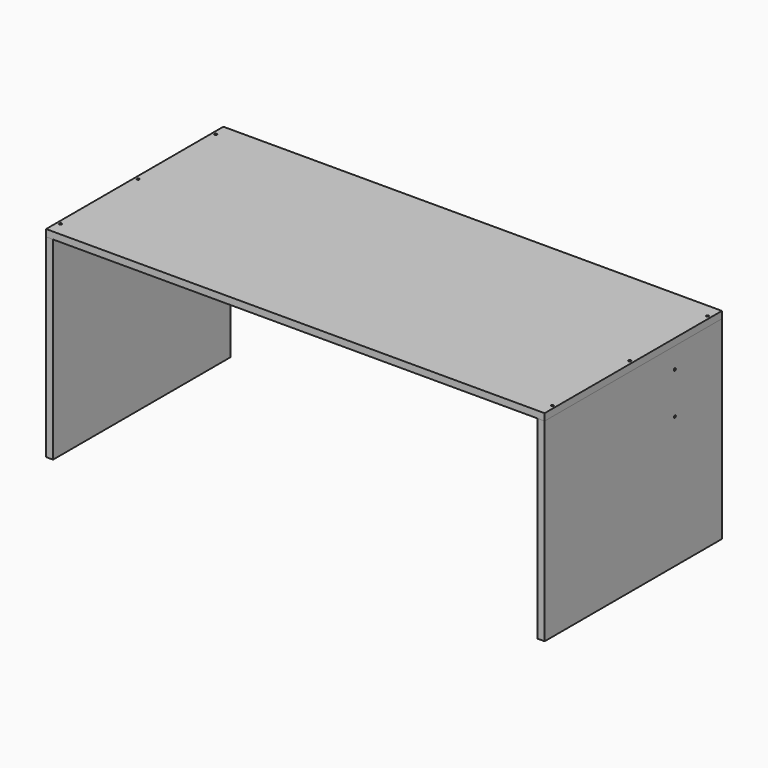
from build123d import *

# Parameters (mm, degrees)
F1_DEPTH          = 800
F0_W              = 25
F0_H              = 700
F2_DEPTH          = 800
F3_W              = 1750
F3_H              = 25
F4_DEPTH          = 300
F6_D              = 4
F6_DEPTH          = 50
F6_CSINK_D        = 8.96
F6_CSINK_ANGLE    = 90
F6_TIP            = 1.2017212381
F6_2_D            = 4
F6_2_DEPTH        = 50
F6_2_CSINK_D      = 8.96
F6_2_CSINK_ANGLE  = 90
F6_2_TIP          = 1.2017212381
F6_3_D            = 4
F6_3_DEPTH        = 50
F6_3_CSINK_D      = 8.96
F6_3_CSINK_ANGLE  = 90
F6_3_TIP          = 1.2017212381
F8_D              = 4
F8_DEPTH          = 40
F8_CSINK_D        = 8.96
F8_CSINK_ANGLE    = 90
F8_TIP            = 1.2017212381
F8_2_D            = 4
F8_2_DEPTH        = 40
F8_2_CSINK_D      = 8.96
F8_2_CSINK_ANGLE  = 90
F8_2_TIP          = 1.2017212381
F10_D             = 4
F10_DEPTH         = 40
F10_CSINK_D       = 8.96
F10_CSINK_ANGLE   = 90
F10_TIP           = 1.2017212381
F10_2_D           = 4
F10_2_DEPTH       = 40
F10_2_CSINK_D     = 8.96
F10_2_CSINK_ANGLE = 90
F10_2_TIP         = 1.2017212381
F12_D             = 3
F12_DEPTH         = 1
F12_TIP           = 0.9012909285
F12_2_D           = 3
F12_2_DEPTH       = 1
F12_2_TIP         = 0.9012909285


# Not quite as in the source:
# - a feature names something its author has since deleted; it is built from what else it names


with BuildPart() as f1:
    # F0 (on Front) → F1 (new body)
    with BuildSketch(Plane.XZ):
        Polygon((0, 25), (0, 0), (25, 0), (1775, 0), (1800, 0), (1800, 25), align=None)
    extrude(amount=-F1_DEPTH)

    # F6
    with Locations(Plane.XY.offset(25)):
        with Locations((12.5, 750), (12.5, 400), (12.5, 50), (1787.5, 750), (1787.5, 400), (1787.5, 50)):
            CounterSinkHole(F6_D / 2, F6_CSINK_D / 2, depth=F6_DEPTH, counter_sink_angle=F6_CSINK_ANGLE)
            with Locations((0, 0, -(F6_DEPTH + F6_TIP / 2))):  # 118° drill point
                Cone(0, F6_D / 2, F6_TIP, mode=Mode.SUBTRACT)


with BuildPart() as f2:
    # F0 (on Front) → F2 (new body)
    with BuildSketch(Plane.XZ):
        with Locations((12.5, -350)):
            Rectangle(F0_W, F0_H)
    extrude(amount=-F2_DEPTH)

    # F6#2
    with Locations(Plane.XY.offset(25)):
        with Locations((12.5, 750), (12.5, 400), (12.5, 50), (1787.5, 750), (1787.5, 400), (1787.5, 50)):
            CounterSinkHole(F6_2_D / 2, F6_2_CSINK_D / 2, depth=F6_2_DEPTH, counter_sink_angle=F6_2_CSINK_ANGLE)
            with Locations((0, 0, -(F6_2_DEPTH + F6_2_TIP / 2))):  # 118° drill point
                Cone(0, F6_2_D / 2, F6_2_TIP, mode=Mode.SUBTRACT)

    # F8
    with Locations(Plane(origin=(0, 0, 0), x_dir=(0, -1, 0), z_dir=(-1, 0, 0))):
        with Locations((-587.5, -75), (-587.5, -225)):
            CounterSinkHole(F8_D / 2, F8_CSINK_D / 2, depth=F8_DEPTH, counter_sink_angle=F8_CSINK_ANGLE)
            with Locations((0, 0, -(F8_DEPTH + F8_TIP / 2))):  # 118° drill point
                Cone(0, F8_D / 2, F8_TIP, mode=Mode.SUBTRACT)

    # F12
    with Locations(Plane(origin=(0, 0, -700), x_dir=(1, 0, 0), z_dir=(0, 0, -1))):
        with Locations((1787.5, -30), (1787.5, -770), (12.5, -30), (12.5, -770)):
            Hole(F12_D / 2, depth=F12_DEPTH)
            with Locations((0, 0, -(F12_DEPTH + F12_TIP / 2))):  # 118° drill point
                Cone(0, F12_D / 2, F12_TIP, mode=Mode.SUBTRACT)


with BuildPart() as f2b:
    # F0 (on Front) → F2, piece 2 (new body)
    with BuildSketch(Plane.XZ):
        with Locations((1787.5, -350)):
            Rectangle(F0_W, F0_H)
    extrude(amount=-F2_DEPTH)

    # F6#3
    with Locations(Plane.XY.offset(25)):
        with Locations((12.5, 750), (12.5, 400), (12.5, 50), (1787.5, 750), (1787.5, 400), (1787.5, 50)):
            CounterSinkHole(F6_3_D / 2, F6_3_CSINK_D / 2, depth=F6_3_DEPTH, counter_sink_angle=F6_3_CSINK_ANGLE)
            with Locations((0, 0, -(F6_3_DEPTH + F6_3_TIP / 2))):  # 118° drill point
                Cone(0, F6_3_D / 2, F6_3_TIP, mode=Mode.SUBTRACT)

    # F10
    with Locations(Plane.YZ.offset(1800)):
        with Locations((587.5, -75), (587.5, -225)):
            CounterSinkHole(F10_D / 2, F10_CSINK_D / 2, depth=F10_DEPTH, counter_sink_angle=F10_CSINK_ANGLE)
            with Locations((0, 0, -(F10_DEPTH + F10_TIP / 2))):  # 118° drill point
                Cone(0, F10_D / 2, F10_TIP, mode=Mode.SUBTRACT)

    # F12#2
    with Locations(Plane(origin=(0, 0, -700), x_dir=(1, 0, 0), z_dir=(0, 0, -1))):
        with Locations((1787.5, -30), (1787.5, -770), (12.5, -30), (12.5, -770)):
            Hole(F12_2_D / 2, depth=F12_2_DEPTH)
            with Locations((0, 0, -(F12_2_DEPTH + F12_2_TIP / 2))):  # 118° drill point
                Cone(0, F12_2_D / 2, F12_2_TIP, mode=Mode.SUBTRACT)


with BuildPart() as f4:
    # F3 (on face) → F4 (new body)
    with BuildSketch(Plane(origin=(0, 0, 0), x_dir=(1, 0, 0), z_dir=(0, 0, -1))):
        with Locations((900, -587.5)):
            Rectangle(F3_W, F3_H)
    extrude(amount=F4_DEPTH)

    # F8#2
    with Locations(Plane(origin=(0, 0, 0), x_dir=(0, -1, 0), z_dir=(-1, 0, 0))):
        with Locations((-587.5, -75), (-587.5, -225)):
            CounterSinkHole(F8_2_D / 2, F8_2_CSINK_D / 2, depth=F8_2_DEPTH, counter_sink_angle=F8_2_CSINK_ANGLE)
            with Locations((0, 0, -(F8_2_DEPTH + F8_2_TIP / 2))):  # 118° drill point
                Cone(0, F8_2_D / 2, F8_2_TIP, mode=Mode.SUBTRACT)

    # F10#2
    with Locations(Plane.YZ.offset(1800)):
        with Locations((587.5, -75), (587.5, -225)):
            CounterSinkHole(F10_2_D / 2, F10_2_CSINK_D / 2, depth=F10_2_DEPTH, counter_sink_angle=F10_2_CSINK_ANGLE)
            with Locations((0, 0, -(F10_2_DEPTH + F10_2_TIP / 2))):  # 118° drill point
                Cone(0, F10_2_D / 2, F10_2_TIP, mode=Mode.SUBTRACT)


solid = Compound([f1.part, f2.part, f2b.part, f4.part])
